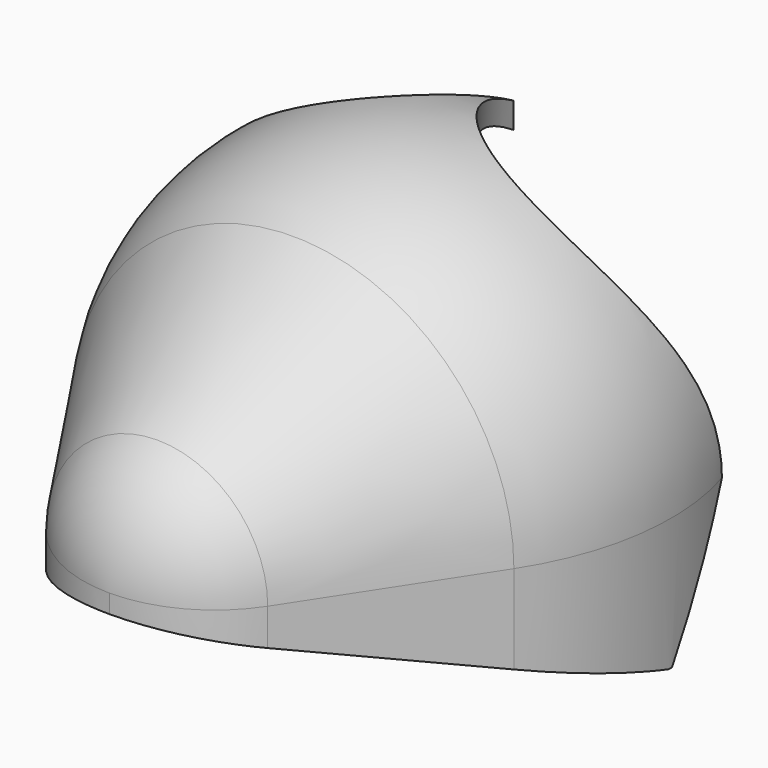
from build123d import *

# Parameters (mm, degrees)
F1_ANGLE = 180
F2_DEPTH = 76.201
F3_DEPTH = 38.1
F5_DEPTH = 127


# Not quite as in the source:
# - a feature names something its author has since deleted; it is built from what else it names


with BuildPart() as f1:
    # F0 (on Top) → F1 (revolve)
    with BuildSketch(Plane.XY):
        with BuildLine():
            ThreePointArc((0, 69.85), (43.8400236241, 54.3789925306), (68.2598802346, 14.819286432))
            ThreePointArc((68.2598802346, 14.819286432), (70.7649049458, 18.4884221725), (72.8257812379, 22.4242187621))
            ThreePointArc((72.8257812379, 22.4242187621), (45.2643045364, 61.299125074), (0, 76.2))
            Line((0, 76.2), (0, 69.85))
        make_face()
        with BuildLine():
            Line((58.5441073038, -38.1), (26.6109578654, -87.1681818182))
            ThreePointArc((26.6109578654, -87.1681818182), (15.1362186043, -97.7598080675), (0, -101.6))
            Line((0, -101.6), (0, -107.95))
            ThreePointArc((0, -107.95), (18.1634623251, -103.341769681), (31.9331494384, -90.6318181818))
            Line((31.9331494384, -90.6318181818), (63.8662988769, -41.5636363636))
            ThreePointArc((63.8662988769, -41.5636363636), (75.4638495733, -10.5663336866), (72.8257812379, 22.4242187621))
            ThreePointArc((72.8257812379, 22.4242187621), (70.7649049458, 18.4884221725), (68.2598802346, 14.819286432))
            ThreePointArc((68.2598802346, 14.819286432), (68.7017141928, -12.6133646173), (58.5441073038, -38.1))
        make_face()
    revolve(axis=Axis((0, -12.7, 0), (0, -1, 0)), revolution_arc=F1_ANGLE)

    # F0 (on Top) → F2 (cut, through all)
    with BuildSketch(Plane.XY):
        with BuildLine():
            ThreePointArc((0, 38.1), (25.8012487817, 2.0396239832), (68.2598802346, 14.819286432))
            ThreePointArc((68.2598802346, 14.819286432), (43.8400236241, 54.3789925306), (0, 69.85))
            Line((0, 69.85), (0, 76.2))
            ThreePointArc((0, 76.2), (45.2643045364, 61.299125074), (72.8257812379, 22.4242187621))
            ThreePointArc((72.8257812379, 22.4242187621), (70.1066966834, 58.7683663461), (38.1, 76.2))
            ThreePointArc((38.1, 76.2), (0, 114.3), (-38.1, 76.2))
            ThreePointArc((-38.1, 76.2), (-65.0407683632, 11.1592316368), (0, 38.1))
        make_face()
        with BuildLine():
            ThreePointArc((0, 69.85), (43.8400236241, 54.3789925306), (68.2598802346, 14.819286432))
            ThreePointArc((68.2598802346, 14.819286432), (70.7649049458, 18.4884221725), (72.8257812379, 22.4242187621))
            ThreePointArc((72.8257812379, 22.4242187621), (45.2643045364, 61.299125074), (0, 76.2))
            Line((0, 76.2), (0, 69.85))
        make_face()
    extrude(amount=F2_DEPTH, mode=Mode.SUBTRACT)

    # F3 (add): a face of the model
    f3_faces = [f1.faces().sort_by_distance(p)[0] for p in [
        (72.4843753918, 17.4560748099, 0),
    ]]
    extrude(f3_faces, amount=F3_DEPTH)

    # F4 (on Right) → F5 (cut, symmetric)
    with BuildSketch(Plane.YZ):
        Polygon((22.4127881229, 0), (0, -38.3907258511), (-2.2853469058, -42.3052824003), (29.7282127851, -42.3052824003), (29.7282127851, 12.5305455596), align=None)
        Polygon((-125.4685521126, -38.3907258511), (0, -38.3907258511), (-125.4685521126, 0), align=None)
    extrude(amount=F5_DEPTH, both=True, mode=Mode.SUBTRACT)


solid = f1.part
